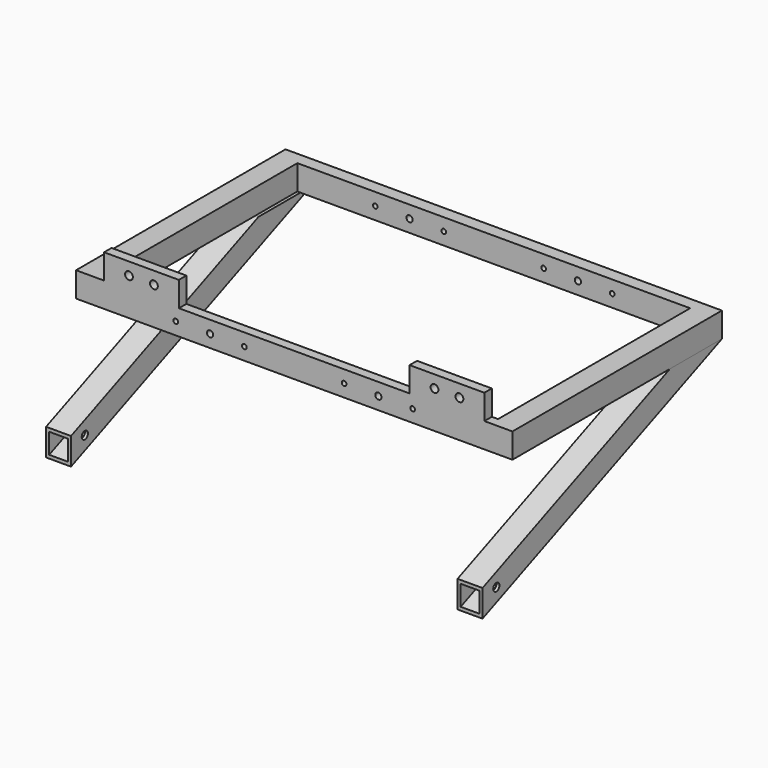
from build123d import *

# Parameters (mm, degrees)
F0_W      = 444.5
F0_H      = 19.05
F1_DEPTH  = 50.8
F2_W      = 152.4
F2_H      = 19.05
F3_DEPTH  = 50.8
F4_W      = 44.45
F4_H      = 50.8
F4_W_2    = 25.4
F4_H_2    = 31.75
F5_DEPTH  = 488.95
F6_W      = 444.5
F6_H      = 50.8
F7_DEPTH  = 25.4
F9_DEPTH  = 25.4
F10_R     = 6.35
F11_DEPTH = 25.4
F13_DEPTH = 50.8
F14_T     = -6.35
F16_DEPTH = 444.501
F17_DEPTH = 444.501
F19_R     = 6.35
F20_DEPTH = 25.4
F18_R     = 4.7625
F21_DEPTH = 609.601


with BuildPart() as f1:
    # F0 (on Top) → F1 (new body)
    with BuildSketch(Plane.XY):
        with Locations((222.25, 9.525)):
            Rectangle(F0_W, F0_H)
    extrude(amount=F1_DEPTH)

    # F2 (on face) → F3 (join)
    with BuildSketch(Plane.XY.offset(50.8)):
        with Locations((311.15, 9.525)):
            Rectangle(F2_W, F2_H)
    extrude(amount=F3_DEPTH)

    # F4 (on face) → F5 (join)
    with BuildSketch(Plane(origin=(0, 19.05, 0), x_dir=(-1, 0, 0), z_dir=(0, 1, 0))):
        with Locations((-422.275, 25.4)):
            Rectangle(F4_W, F4_H)
        with Locations((-422.275, 25.4)):
            Rectangle(F4_W_2, F4_H_2, mode=Mode.SUBTRACT)
    extrude(amount=F5_DEPTH)

    # F6 (on face) → F7 (join)
    with BuildSketch(Plane(origin=(0, 508, 0), x_dir=(-1, 0, 0), z_dir=(0, 1, 0))):
        with Locations((-222.25, 25.4)):
            Rectangle(F6_W, F6_H)
    extrude(amount=F7_DEPTH)

    # F8 (on face) → F9 (cut)
    with BuildSketch(Plane(origin=(0, 19.05, 0), x_dir=(-1, 0, 0), z_dir=(0, 1, 0))):
        with BuildLine():
            ThreePointArc((-328.6125, 76.2), (-336.55, 84.1375), (-344.4875, 76.2))
            Line((-344.4875, 76.2), (-336.55, 76.2))
            Line((-336.55, 76.2), (-328.6125, 76.2))
        make_face()
        with BuildLine():
            ThreePointArc((-277.8125, 76.2), (-285.75, 84.1375), (-293.6875, 76.2))
            ThreePointArc((-293.6875, 76.2), (-285.75, 68.2625), (-277.8125, 76.2))
        make_face()
        with BuildLine():
            Line((-336.55, 76.2), (-344.4875, 76.2))
            ThreePointArc((-344.4875, 76.2), (-336.55, 68.2625), (-328.6125, 76.2))
            Line((-328.6125, 76.2), (-336.55, 76.2))
        make_face()
    extrude(amount=-F9_DEPTH, mode=Mode.SUBTRACT)

    # F10 (on face) → F11 (cut)
    with BuildSketch(Plane.XZ):
        with Locations((171.45, 25.4)):
            Circle(F10_R)
    extrude(amount=-F11_DEPTH, mode=Mode.SUBTRACT)

    # F15 (on face) → F17 (cut, through all)
    with BuildSketch(Plane.YZ.offset(444.5)):
        with BuildLine():
            ThreePointArc((-33.7038461538, -208.7766025641), (-44.0836538462, -204.5025641026), (-48.3576923077, -214.8823717949))
            Line((-48.3576923077, -214.8823717949), (-33.7038461538, -208.7766025641))
        make_face()
        with BuildLine():
            Line((-33.7038461538, -208.7766025641), (-48.3576923077, -214.8823717949))
            ThreePointArc((-48.3576923077, -214.8823717949), (-39.4740974081, -219.6128462928), (-33.0932692308, -211.8294871795))
            ThreePointArc((-33.0932692308, -211.8294871795), (-33.2474101175, -210.2728153568), (-33.7038461538, -208.7766025641))
        make_face()
    extrude(amount=-F17_DEPTH, mode=Mode.SUBTRACT)

    # F19 (on face) → F20 (cut)
    with BuildSketch(Plane.XZ.offset(-508)):
        with Locations((171.45, 25.4)):
            Circle(F19_R)
    extrude(amount=-F20_DEPTH, mode=Mode.SUBTRACT)

    # F18 (on face) → F21 (cut, through all)
    with BuildSketch(Plane(origin=(0, 533.4, 0), x_dir=(-1, 0, 0), z_dir=(0, 1, 0))):
        with Locations((-241.3, 25.4)):
            Circle(F18_R)
        with Locations((-101.6, 25.4)):
            Circle(F18_R)
    extrude(amount=-F21_DEPTH, mode=Mode.SUBTRACT)



with BuildPart() as f13:
    # F12 (on face) → F13 (new body)
    with BuildSketch(Plane.YZ.offset(444.5)):
        Polygon((401.32, 0), (-76.2, -198.9666666667), (-76.2, -254), (533.4, 0), align=None)
    extrude(amount=-F13_DEPTH)

    # F14
    f14_openings = [f13.faces().sort_by_distance(p)[0] for p in [
        (419.1, -76.2, -226.483333),
    ]]
    offset(amount=F14_T, openings=f14_openings)

    # F15 (on face) → F16 (cut, through all)
    with BuildSketch(Plane.YZ.offset(444.5)):
        with BuildLine():
            ThreePointArc((-33.7038461538, -208.7766025641), (-44.0836538462, -204.5025641026), (-48.3576923077, -214.8823717949))
            Line((-48.3576923077, -214.8823717949), (-33.7038461538, -208.7766025641))
        make_face()
        with BuildLine():
            Line((-33.7038461538, -208.7766025641), (-48.3576923077, -214.8823717949))
            ThreePointArc((-48.3576923077, -214.8823717949), (-39.4740974081, -219.6128462928), (-33.0932692308, -211.8294871795))
            ThreePointArc((-33.0932692308, -211.8294871795), (-33.2474101175, -210.2728153568), (-33.7038461538, -208.7766025641))
        make_face()
    extrude(amount=-F16_DEPTH, mode=Mode.SUBTRACT)


with BuildPart() as f1_1:
    add(f1.part)
    # F22: F13, F1 across plane
    add(f13.part.mirror(Plane.YZ))
    add(f1.part.mirror(Plane.YZ))


solid = Compound([f13.part, f1_1.part])
